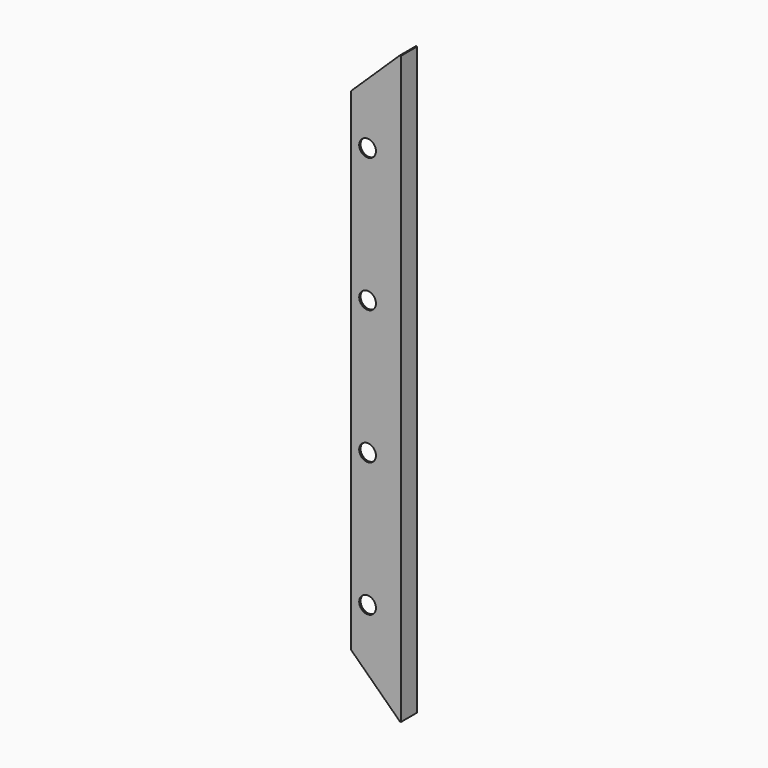
from build123d import *

# Parameters (mm, degrees)
F1_DEPTH = 3500
F3_DEPTH = 200
F4_R     = 50
F5_DEPTH = 120.001


# Not quite as in the source:
# - a feature names something its author has since deleted; it is built from what else it names


with BuildPart() as f1:
    # F0 (on Top) → F1 (new body)
    with BuildSketch(Plane.XY):
        Polygon((-100, 0), (-110, 0), (-110, -30), (190, -30), (190, 90), (180, 90), (180, -20), (-100, -20), align=None)
    extrude(amount=F1_DEPTH)

    # F2 (on face) → F3 (cut)
    with BuildSketch(Plane.XZ.offset(30)):
        Polygon((182.8939372419, 0), (-110, 282.8443874035), (-110, 0), align=None)
        Polygon((-110, 3500), (-110, 3217.1556125965), (182.8939372419, 3500), align=None)
    extrude(amount=-F3_DEPTH, mode=Mode.SUBTRACT)

    # F4 (on face) → F5 (cut, through all)
    with BuildSketch(Plane.XZ.offset(30)):
        with Locations((-10, 2950)):
            Circle(F4_R)
        with Locations((-10, 2150)):
            Circle(F4_R)
        with Locations((-10, 1350)):
            Circle(F4_R)
        with Locations((-10, 550)):
            Circle(F4_R)
    extrude(amount=-F5_DEPTH, mode=Mode.SUBTRACT)


solid = f1.part
